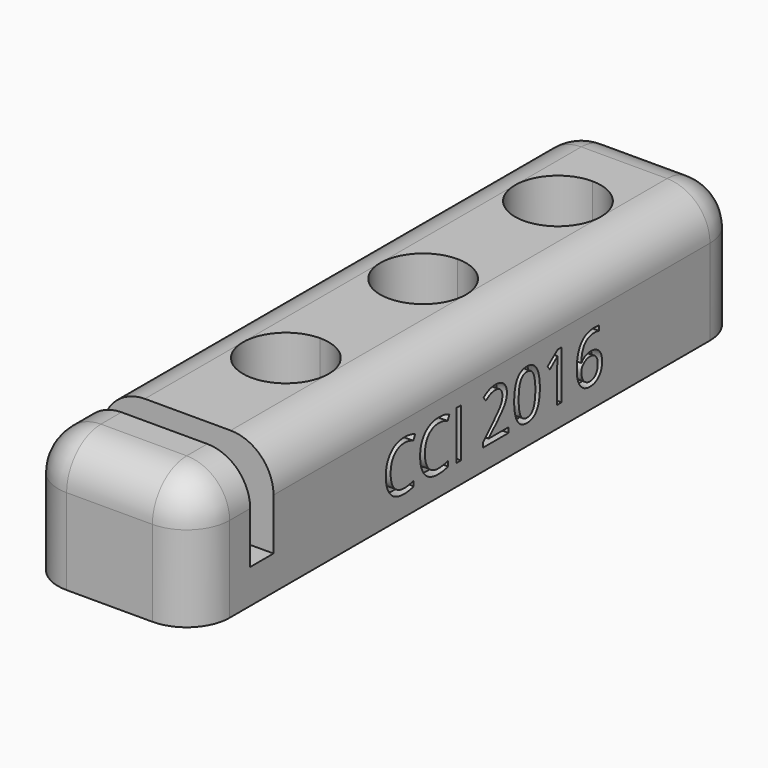
from build123d import *

# Parameters (mm, degrees)
F0_W         = 20
F0_H         = 80
F1_DEPTH     = 15
F3_DEPTH     = 11
F4_DEPTH     = 25
F5_R         = 5
F6_R         = 4.99999
F7_TEXT_SIZE = 7.9238214918
F8_DEPTH     = 1.2


# Not quite as in the source:
# - a fillet or chamfer is up to 0.001 mm smaller than in the source, because OpenCascade refuses the exact size
# - Text() gives the source's letters only with a copy of the font that has no kerning and outlines rounded to 1/6400 em; it was checked with that copy


with BuildPart() as f1:
    # F0 (on Top) → F1 (new body)
    with BuildSketch(Plane.XY):
        Rectangle(F0_W, F0_H)
    extrude(amount=F1_DEPTH)

    # F2 (on face) → F3 (cut)
    with BuildSketch(Plane.XY.offset(15)):
        Polygon((-10, -28.6), (-10, -32), (10, -32), (10, -28.6), (0, -28.6), align=None)
    extrude(amount=-F3_DEPTH, mode=Mode.SUBTRACT)

    # F2 (on face) → F4 (cut)
    with BuildSketch(Plane.XY.offset(15)):
        with BuildLine():
            ThreePointArc((5, 25.35), (3.5355339059, 28.8855339059), (0, 30.35))
            Line((0, 30.35), (0, 20.35))
            ThreePointArc((0, 20.35), (3.5355339059, 21.8144660941), (5, 25.35))
        make_face()
        with BuildLine():
            Line((0, 20.35), (0, 30.35))
            ThreePointArc((0, 30.35), (-5, 25.35), (0, 20.35))
        make_face()
        with BuildLine():
            Line((0, 10.7), (0, 0.7))
            ThreePointArc((0, 0.7), (3.5355339059, 2.1644660941), (5, 5.7))
            ThreePointArc((5, 5.7), (3.5355339059, 9.2355339059), (0, 10.7))
        make_face()
        with BuildLine():
            ThreePointArc((0, 10.7), (-5, 5.7), (0, 0.7))
            Line((0, 0.7), (0, 10.7))
        make_face()
        with BuildLine():
            ThreePointArc((0, -9.3), (-5, -14.3), (0, -19.3))
            Line((0, -19.3), (0, -9.3))
        make_face()
        with BuildLine():
            Line((0, -9.3), (0, -19.3))
            ThreePointArc((0, -19.3), (3.5355339059, -17.8355339059), (5, -14.3))
            ThreePointArc((5, -14.3), (3.5355339059, -10.7644660941), (0, -9.3))
        make_face()
    extrude(amount=-F4_DEPTH, mode=Mode.SUBTRACT)

    # F5
    f5_edges = [f1.edges().sort_by_distance(p)[0] for p in [
        (-10, 40, 7.5),
        (-10, -40, 7.5),
        (10, -40, 7.5),
        (10, 40, 7.5),
    ]]
    fillet(f5_edges, radius=F5_R)

    # F6 (radius 5 in the source; OpenCascade refuses exactly that, so slightly less here)
    f6_edges = [f1.edges().sort_by_distance(p)[0] for p in [
        (-10, 3.2, 15),
        (8.535534, -38.535534, 15),
    ]]
    fillet(f6_edges, radius=F6_R)

    # F7 (on face) → F8 (cut)
    with BuildSketch(Plane.YZ.offset(10)):
        with Locations((-12.7205784083, 2.4507360067)):
            Text('CCI 2016', F7_TEXT_SIZE, font='Open Sans', text_align=(TextAlign.LEFT, TextAlign.BOTTOM))
    extrude(amount=-F8_DEPTH, mode=Mode.SUBTRACT)


solid = f1.part
